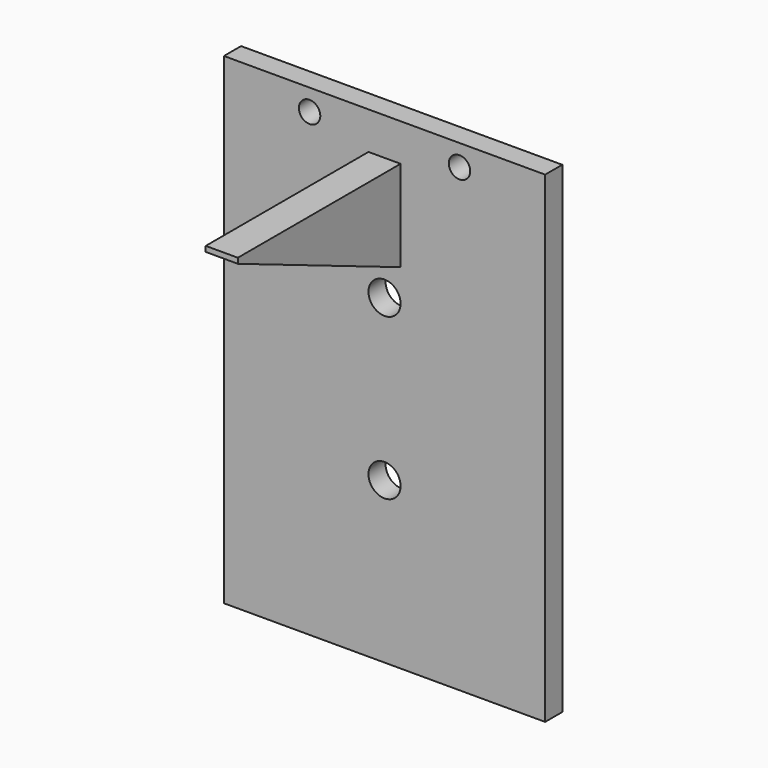
from build123d import *

# Parameters (mm, degrees)
F0_W     = 30
F0_H     = 45
F1_DEPTH = 2
F3_D     = 2
F4_D     = 3
F2_W     = 3
F2_H     = 8.5
F5_DEPTH = 19
F6_SIZE2 = 18.99999
F6_SIZE  = 7.99999


# Not quite as in the source:
# - a fillet or chamfer is up to 0.001 mm smaller than in the source, because OpenCascade refuses the exact size


with BuildPart() as f1:
    # F0 (on Front) → F1 (new body)
    with BuildSketch(Plane.XZ):
        Rectangle(F0_W, F0_H)
    extrude(amount=F1_DEPTH)

    # F3 (through all)
    with Locations(Plane.XZ.offset(2)):
        with Locations((-7, 20.5), (7, 20.5)):
            Hole(F3_D / 2)

    # F4 (through all)
    with Locations(Plane.XZ.offset(2)):
        with Locations((0, 7.5), (0, -7.5)):
            Hole(F4_D / 2)

    # F2 (on face) → F5 (join)
    with BuildSketch(Plane.XZ.offset(2)):
        with Locations((0, 14.75)):
            Rectangle(F2_W, F2_H)
    extrude(amount=F5_DEPTH)

    # F6 (size 8 and 19 in the source; OpenCascade refuses exactly that, so slightly less here)
    f6_edges = [f1.edges().sort_by_distance(p)[0] for p in [
        (0, -21, 10.5),
    ]]
    f6_side = f1.faces().sort_by_distance((0, -21, 14.75))[0]
    chamfer(f6_edges, length=F6_SIZE, length2=F6_SIZE2, reference=f6_side)


solid = f1.part
